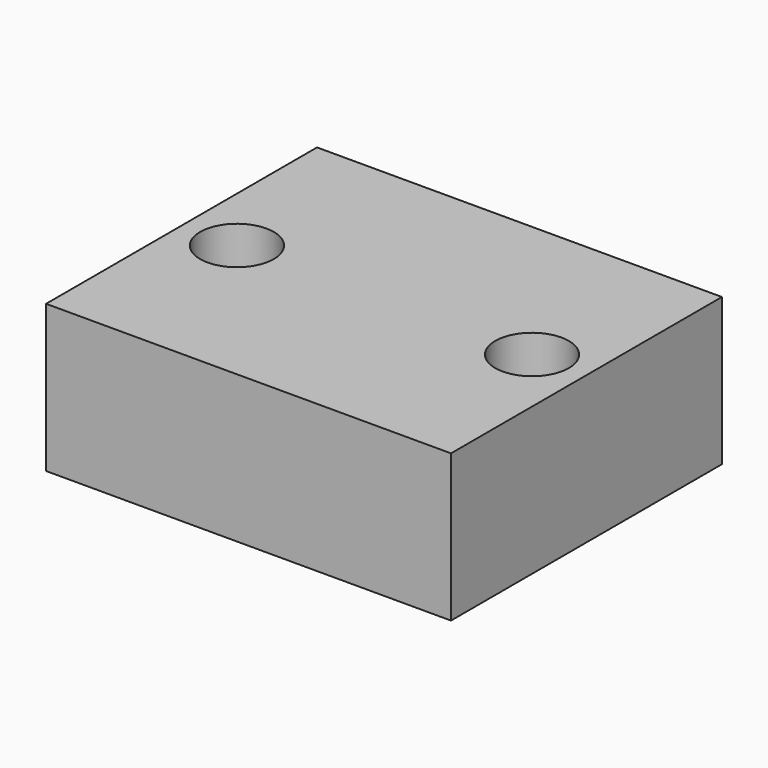
from build123d import *

# Parameters (mm, degrees)
F0_W     = 139.7
F0_H     = 116.84
F0_R     = 12.7
F1_DEPTH = 50.8


# Not quite as in the source:
# - the program builds the solid bodies; features that only make, move or delete a surface that nothing else refers to are left out


with BuildPart() as f1:
    # F0 (on Top) → F1 (new body)
    with BuildSketch(Plane.XY):
        with Locations((-10.3572173724, -0.2563824468)):
            Rectangle(F0_W, F0_H)
        with Locations((-61.2939819694, 0)):
            Circle(F0_R, mode=Mode.SUBTRACT)
        with BuildLine():
            ThreePointArc((27.8118101201, 0), (40.5118101201, 12.7), (53.2118101201, 0))
            ThreePointArc((53.2118101201, 0), (40.5118101201, -12.7), (27.8118101201, 0))
        make_face(mode=Mode.SUBTRACT)
    extrude(amount=-F1_DEPTH)


solid = f1.part
